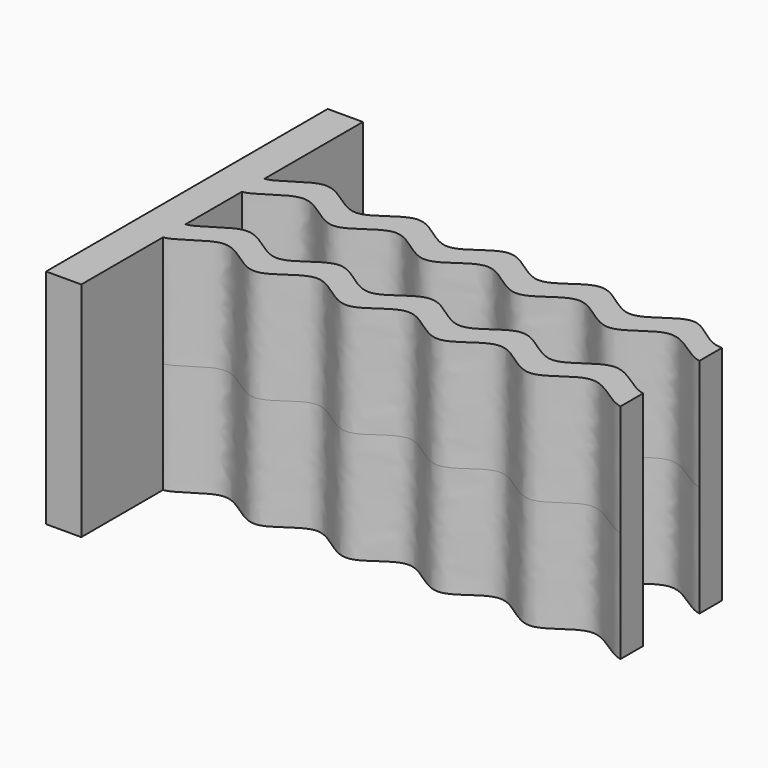
from build123d import *

# Parameters (mm, degrees)
F1_DEPTH = 7.9


with BuildPart() as f1:
    # F0 (on Top) → F1 (new body, symmetric)
    with BuildSketch(Plane.XY):
        with BuildLine():
            Line((-32.5, 20.0030848121), (-35, 20.0030848121))
            Line((-35, 20.0030848121), (-35, 12.7530848121))
            add(Edge.make_bspline(
                [(-35, 12.7530848121), (-34.2035043996, 11.9260806463), (-33.4070087991, 11.0990764805), (-32.5, 11.2530848121)],
                knots=[0, 0, 0, 0, 0.0754165891, 0.0754165891, 0.0754165891, 0.0754165891], degree=3))
            Line((-32.5, 11.2530848121), (-32.5, 20.0030848121))
        make_face()
        with BuildLine():
            add(Edge.make_bspline(
                [(-35, 12.7530848121), (-34.2035043996, 11.9260806463), (-33.4070087991, 11.0990764805), (-32.5, 11.2530848121)],
                knots=[0, 0, 0, 0, 0.0754165891, 0.0754165891, 0.0754165891, 0.0754165891], degree=3))
            Line((-35, 12.7530848121), (-35, 10.7530848121))
            add(Edge.make_bspline(
                [(-35, 10.7530848121), (-34.2035042168, 9.9260808378), (-33.4070084337, 9.0990768636), (-32.5, 9.2530848121)],
                knots=[0, 0, 0, 0, 0.0760556357, 0.0760556357, 0.0760556357, 0.0760556357], degree=3))
            Line((-32.5, 9.2530848121), (-32.5, 11.2530848121))
        make_face()
        with BuildLine():
            add(Edge.make_bspline(
                [(-32.5, 11.2530848121), (-31.4950019052, 11.4237315357), (-29.2136420975, 14.1738874896), (-26.009749801, 9.7743053553), (-22.7473586987, 14.2473999618), (-19.5008154044, 9.75460367), (-16.2493796837, 14.2526942305), (-13.0016658609, 9.7531282803), (-9.7439568726, 14.2533015207), (-6.5225066486, 9.7521745093), (-3.1660165331, 14.2565093144), (-1.2642903237, 11.2457011751), (0, 11.2530848121)],
                knots=[0.0754165891, 0.0754165891, 0.0754165891, 0.0754165891, 0.1589808592, 0.2425451294, 0.3261093996, 0.4096736697, 0.4932379399, 0.5768022101, 0.6603664802, 0.7439307504, 0.8274950205, 0.9110592907, 0.9110592907, 0.9110592907, 0.9110592907], degree=3))
            Line((-32.5, 11.2530848121), (-32.5, 9.2530848121))
            add(Edge.make_bspline(
                [(-32.5, 9.2530848121), (-31.4950023101, 9.4237311112), (-29.2136446583, 12.1738848053), (-26.0097402308, 7.7743153872), (-22.7473944185, 12.2473625184), (-19.5006820954, 7.7547434118), (-16.2498772001, 12.252172707), (-12.9998091044, 7.7550746328), (-9.7508863824, 12.2460376344), (-6.4966453659, 7.779283702), (-3.2625321541, 12.1553364301), (-1.0563280632, 9.4636984435), (0, 9.2530848121)],
                knots=[0.0760556357, 0.0760556357, 0.0760556357, 0.0760556357, 0.1603279924, 0.244600349, 0.3288727057, 0.4131450623, 0.497417419, 0.5816897756, 0.6659621323, 0.7502344889, 0.8345068456, 0.9187792022, 0.9187792022, 0.9187792022, 0.9187792022], degree=3))
            Line((0, 9.2530848121), (0, 11.2530848121))
        make_face()
        with BuildLine():
            add(Edge.make_bspline(
                [(-35, 10.7530848121), (-34.2035042168, 9.9260808378), (-33.4070084337, 9.0990768636), (-32.5, 9.2530848121)],
                knots=[0, 0, 0, 0, 0.0760556357, 0.0760556357, 0.0760556357, 0.0760556357], degree=3))
            Line((-35, 10.7530848121), (-35, 5.7530848121))
            add(Edge.make_bspline(
                [(-35, 5.7530848121), (-34.2035042168, 4.9260808378), (-33.4070084337, 4.0990768636), (-32.5, 4.2530848121)],
                knots=[0, 0, 0, 0, 0.0760556357, 0.0760556357, 0.0760556357, 0.0760556357], degree=3))
            Line((-32.5, 4.2530848121), (-32.5, 9.2530848121))
        make_face()
        with BuildLine():
            add(Edge.make_bspline(
                [(-35, 5.7530848121), (-34.2035042168, 4.9260808378), (-33.4070084337, 4.0990768636), (-32.5, 4.2530848121)],
                knots=[0, 0, 0, 0, 0.0760556357, 0.0760556357, 0.0760556357, 0.0760556357], degree=3))
            Line((-35, 5.7530848121), (-35, 3.7530848121))
            add(Edge.make_bspline(
                [(-35, 3.7530848121), (-34.2035042168, 2.9260808378), (-33.4070084337, 2.0990768636), (-32.5, 2.2530848121)],
                knots=[0, 0, 0, 0, 0.0760556357, 0.0760556357, 0.0760556357, 0.0760556357], degree=3))
            Line((-32.5, 2.2530848121), (-32.5, 4.2530848121))
        make_face()
        with BuildLine():
            add(Edge.make_bspline(
                [(-32.5, 4.2530848121), (-31.4950023101, 4.4237311112), (-29.2136446583, 7.1738848053), (-26.0097402308, 2.7743153872), (-22.7473944185, 7.2473625184), (-19.5006820954, 2.7547434118), (-16.2498772001, 7.252172707), (-12.9998091044, 2.7550746328), (-9.7508863824, 7.2460376344), (-6.4966453659, 2.779283702), (-3.2625321541, 7.1553364301), (-1.0563280632, 4.4636984435), (0, 4.2530848121)],
                knots=[0.0760556357, 0.0760556357, 0.0760556357, 0.0760556357, 0.1603279924, 0.244600349, 0.3288727057, 0.4131450623, 0.497417419, 0.5816897756, 0.6659621323, 0.7502344889, 0.8345068456, 0.9187792022, 0.9187792022, 0.9187792022, 0.9187792022], degree=3))
            Line((-32.5, 4.2530848121), (-32.5, 2.2530848121))
            add(Edge.make_bspline(
                [(-32.5, 2.2530848121), (-31.4950023101, 2.4237311112), (-29.2136446583, 5.1738848053), (-26.0097402308, 0.7743153872), (-22.7473944185, 5.2473625184), (-19.5006820954, 0.7547434118), (-16.2498772001, 5.252172707), (-12.9998091044, 0.7550746328), (-9.7508863824, 5.2460376344), (-6.4966453659, 0.779283702), (-3.2625321541, 5.1553364301), (-1.0563280632, 2.4636984435), (0, 2.2530848121)],
                knots=[0.0760556357, 0.0760556357, 0.0760556357, 0.0760556357, 0.1603279924, 0.244600349, 0.3288727057, 0.4131450623, 0.497417419, 0.5816897756, 0.6659621323, 0.7502344889, 0.8345068456, 0.9187792022, 0.9187792022, 0.9187792022, 0.9187792022], degree=3))
            Line((0, 2.2530848121), (0, 4.2530848121))
        make_face()
        with BuildLine():
            add(Edge.make_bspline(
                [(-35, 3.7530848121), (-34.2035042168, 2.9260808378), (-33.4070084337, 2.0990768636), (-32.5, 2.2530848121)],
                knots=[0, 0, 0, 0, 0.0760556357, 0.0760556357, 0.0760556357, 0.0760556357], degree=3))
            Line((-35, 3.7530848121), (-35, -4.9969151879))
            Line((-35, -4.9969151879), (-32.5, -4.9969151879))
            Line((-32.5, -4.9969151879), (-32.5, 2.2530848121))
        make_face()
    extrude(amount=F1_DEPTH, both=True)


solid = f1.part
